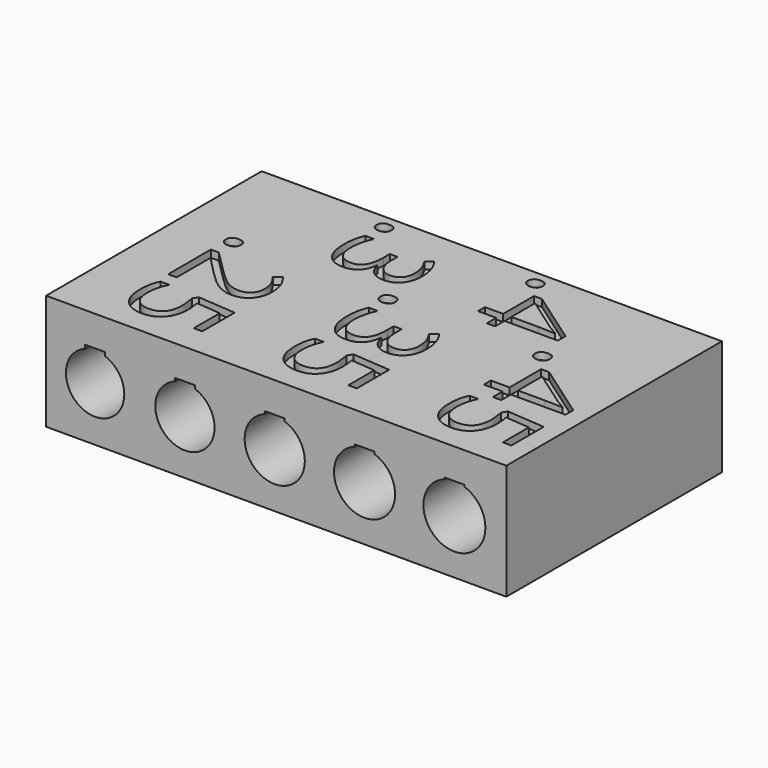
from build123d import *

# Parameters (mm, degrees)
F0_W           = 25.6193375681
F0_H           = 6.4234328456
F1_DEPTH       = 15
F2_TEXT_SIZE   = 6.3256313327
F2_TEXT_SIZE_2 = 6.1921270369
F3_DEPTH       = 0.4


# Not quite as in the source:
# - Text() gives the source's letters only with a copy of the font that has no kerning and outlines rounded to 1/6400 em; it was checked with that copy


with BuildPart() as f1:
    # F0 (on Front) → F1 (new body)
    with BuildSketch(Plane.XZ):
        with Locations((10.0818210049, 3.2117164228)):
            Rectangle(F0_W, F0_H)
        with BuildLine():
            ThreePointArc((0.5496821429, 4.5292071612), (1.3292589067, 3.9347169405), (1.625, 3))
            ThreePointArc((1.625, 3), (-0.9347169405, 1.6707410933), (-0.5496821429, 4.5292071612))
            Line((-0.5496821429, 4.5292071612), (-0.5496821429, 4.7284820447))
            Line((-0.5496821429, 4.7284820447), (0.5496821429, 4.7284820447))
            Line((0.5496821429, 4.7284820447), (0.5496821429, 4.5292071612))
        make_face(mode=Mode.SUBTRACT)
        with BuildLine():
            ThreePointArc((5.5496821429, 4.5557472615), (6.3471220316, 3.9527655704), (6.65, 3))
            ThreePointArc((6.65, 3), (4.0472344296, 1.6528779684), (4.4503178571, 4.5557472615))
            Line((4.4503178571, 4.5557472615), (4.4503178571, 4.7284820447))
            Line((4.4503178571, 4.7284820447), (5.5496821429, 4.7284820447))
            Line((5.5496821429, 4.7284820447), (5.5496821429, 4.5557472615))
        make_face(mode=Mode.SUBTRACT)
        with BuildLine():
            ThreePointArc((10.5496821429, 4.5822371952), (11.3649803276, 3.9708005487), (11.675, 3))
            ThreePointArc((11.675, 3), (9.0291994513, 1.6350196724), (9.4503178571, 4.5822371952))
            Line((9.4503178571, 4.5822371952), (9.4503178571, 4.7284820447))
            Line((9.4503178571, 4.7284820447), (10.5496821429, 4.7284820447))
            Line((10.5496821429, 4.7284820447), (10.5496821429, 4.5822371952))
        make_face(mode=Mode.SUBTRACT)
        with BuildLine():
            ThreePointArc((15.5496821429, 4.6086794403), (16.3828339819, 3.9888226224), (16.7, 3))
            ThreePointArc((16.7, 3), (14.0111773776, 1.6171660181), (14.4503178571, 4.6086794403))
            Line((14.4503178571, 4.6086794403), (14.4503178571, 4.7284820447))
            Line((14.4503178571, 4.7284820447), (15.5496821429, 4.7284820447))
            Line((15.5496821429, 4.7284820447), (15.5496821429, 4.6086794403))
        make_face(mode=Mode.SUBTRACT)
        with BuildLine():
            ThreePointArc((20.5496821429, 4.6350763107), (21.400683172, 4.0068324844), (21.725, 3))
            ThreePointArc((21.725, 3), (18.9931675156, 1.599316828), (19.4503178571, 4.6350763107))
            Line((19.4503178571, 4.6350763107), (19.4503178571, 4.7284820447))
            Line((19.4503178571, 4.7284820447), (20.5496821429, 4.7284820447))
            Line((20.5496821429, 4.7284820447), (20.5496821429, 4.6350763107))
        make_face(mode=Mode.SUBTRACT)
    extrude(amount=-F1_DEPTH)

    # F2 (on face) → F3 (cut)
    with BuildSketch(Plane.XY.offset(6.4234328456)):
        with Locations(Location((17.3587912264, 9.854590576), (0, 0, -90))):
            Text('.45', F2_TEXT_SIZE, font='Open Sans', text_align=(TextAlign.LEFT, TextAlign.BOTTOM))
        with Locations(Location((8.7559326139, 9.854590576), (0, 0, -90))):
            Text('.35', F2_TEXT_SIZE, font='Open Sans', text_align=(TextAlign.LEFT, TextAlign.BOTTOM))
        with Locations(Location((0.1530740014, 9.854590576), (0, 0, -90))):
            Text('.25', F2_TEXT_SIZE, font='Open Sans', text_align=(TextAlign.LEFT, TextAlign.BOTTOM))
        with Locations(Location((12.8403087511, 15), (0, 0, -90))):
            Text('.4', F2_TEXT_SIZE_2, font='Open Sans', text_align=(TextAlign.LEFT, TextAlign.BOTTOM))
        with Locations(Location((4.419015981, 15), (0, 0, -90))):
            Text('.3', F2_TEXT_SIZE_2, font='Open Sans', text_align=(TextAlign.LEFT, TextAlign.BOTTOM))
    extrude(amount=-F3_DEPTH, mode=Mode.SUBTRACT)


solid = f1.part
